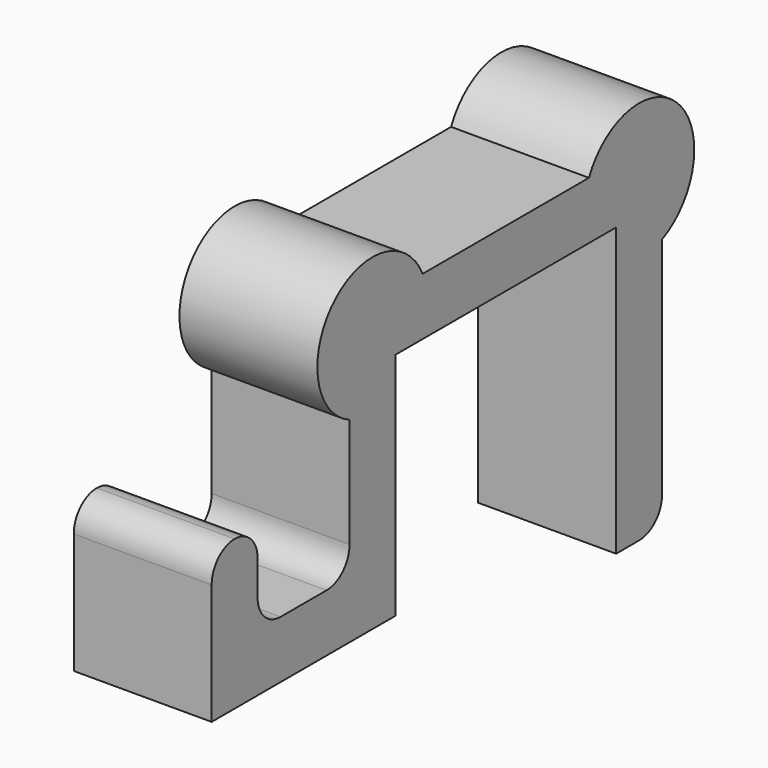
from build123d import *

# Parameters (mm, degrees)
F1_DEPTH = 12
F2_R     = 2.49999


# Not quite as in the source:
# - a fillet or chamfer is up to 0.001 mm smaller than in the source, because OpenCascade refuses the exact size


with BuildPart() as f1:
    # F0 (on Right) → F1 (new body)
    with BuildSketch(Plane.YZ):
        Polygon((-20, 0), (0, 0), (0, 20), (-5, 25), (-5, 17.0456439427), (-5, 5), (-15, 5), (-15, 13), (-20, 13), align=None)
        Polygon((-5, 25), (0, 20), (24, 20), (29, 25), (21.0456439427, 25), (2.9543560573, 25), align=None)
        Polygon((29, 25), (24, 20), (24, -5), (29, -5), (29, 17.0456439427), align=None)
        with BuildLine():
            Line((-5, 17.0456439427), (-5, 25))
            Line((-5, 25), (2.9543560573, 25))
            ThreePointArc((2.9543560573, 25), (-6.7426406871, 26.7426406871), (-5, 17.0456439427))
        make_face()
        with BuildLine():
            Line((21.0456439427, 25), (29, 25))
            Line((29, 25), (29, 17.0456439427))
            ThreePointArc((29, 17.0456439427), (30.7426406871, 26.7426406871), (21.0456439427, 25))
        make_face()
    extrude(amount=F1_DEPTH)

    # F2 (radius 2.5 in the source; OpenCascade refuses exactly that, so slightly less here)
    f2_edges = [f1.edges().sort_by_distance(p)[0] for p in [
        (6, -5, 5),
        (6, -15, 5),
        (6, 29, -5),
        (6, -20, 13),
        (6, -15, 13),
    ]]
    fillet(f2_edges, radius=F2_R)


solid = f1.part
